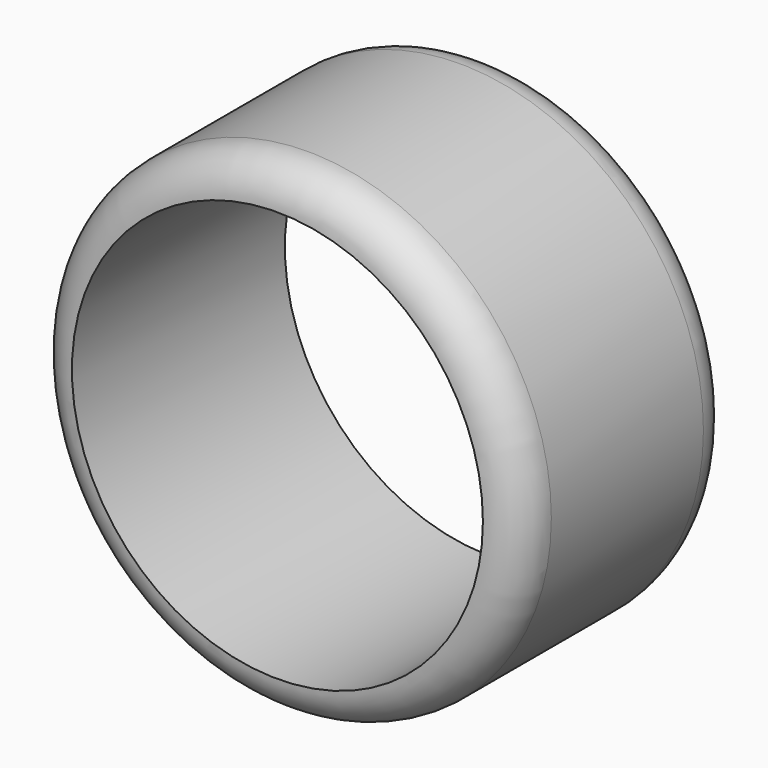
from build123d import *

# Parameters (mm, degrees)
F0_R     = 137.2744361776
F1_DEPTH = 177.8
F2_T     = 25.4


# Not quite as in the source:
# - a fillet or chamfer that OpenCascade refuses, or shapes differently, is made with other operations: its cross-section is extruded or revolved along the edge and cut away or added


with BuildPart() as f1:
    # F0 (on Front) → F1 (new body)
    with BuildSketch(Plane.XZ):
        with Locations((-6.2283538282, -7.7867358923)):
            Circle(F0_R)
    extrude(amount=F1_DEPTH)

    # F2
    f2_openings = [f1.faces().sort_by_distance(p)[0] for p in [
        (-6.228354, -177.8, -7.786736),
        (-6.228354, 0, -7.786736),
    ]]
    offset(amount=F2_T, openings=f2_openings)

    # F3: fillet of radius 25.4 on 2 edges, made by hand

    # F3_s1 → F3_t2 (revolve, cut)
    with BuildSketch(Plane.XY.offset(-7.7867358923)):
        with BuildLine():
            ThreePointArc((131.0460823494, 0), (149.0065945915, -7.4394877579), (156.4460823494, -25.4))
            Line((156.4460823494, -25.4), (156.4460823494, 0))
            Line((156.4460823494, 0), (131.0460823494, 0))
        make_face()
    revolve(axis=Axis((-6.2283538282, 0, -7.7867358923), (0, -1, 0)), mode=Mode.SUBTRACT)

    # F3_s3 → F3_t4 (revolve, cut)
    with BuildSketch(Plane.XY.offset(-7.7867358923)):
        with BuildLine():
            ThreePointArc((156.4460823494, -152.4), (149.0065945915, -170.3605122421), (131.0460823494, -177.8))
            Line((131.0460823494, -177.8), (156.4460823494, -177.8))
            Line((156.4460823494, -177.8), (156.4460823494, -152.4))
        make_face()
    revolve(axis=Axis((-6.2283538282, -177.8, -7.7867358923), (0, -1, 0)), mode=Mode.SUBTRACT)


solid = f1.part
